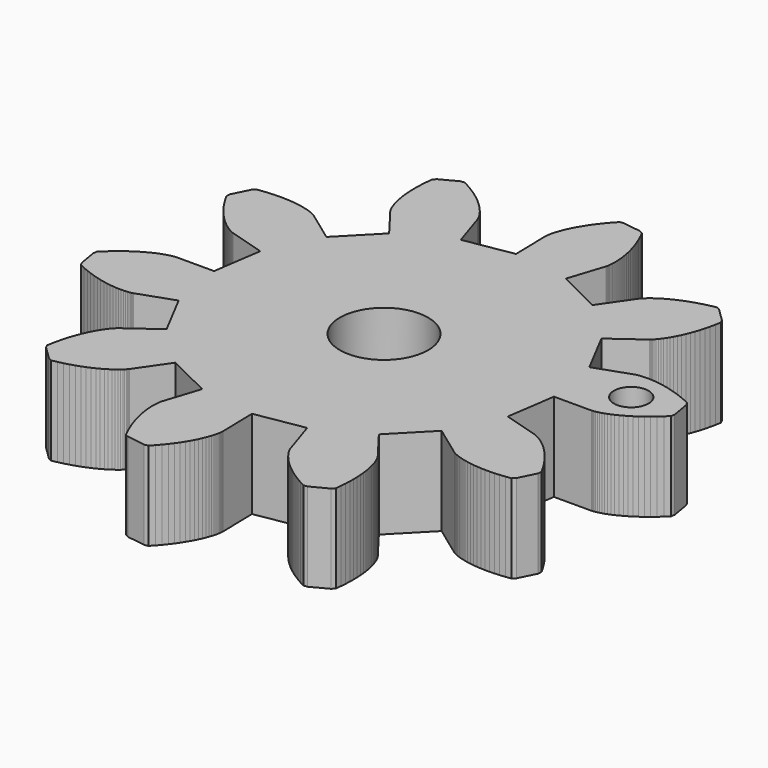
from build123d import *

# Parameters (mm, degrees)
F0_R     = 2.5
F1_DEPTH = 5


# Not quite as in the source:
# - the dataset's text gives a spline's control points without its knots; the knots are read off the source's solid


with BuildPart() as f1:
    # F0 (on Top) → F1 (new body)
    with BuildSketch(Plane.XY):
        Polygon((13.6310377596, 0.7067476629), (14.0365257596, 3.4714366629), (16.1597377596, 3.4714366629), (16.1738627596, 3.4719536629), (16.2024577596, 3.4740206629), (16.2451767596, 3.4784996629), (16.3016757596, 3.4865956629), (16.3723007596, 3.4989976629), (16.4563607596, 3.5169126629), (16.5535127596, 3.5412006629), (16.6634107596, 3.5727226629), (16.7860567596, 3.6126856629), (16.9204147596, 3.6616066629), (17.0664877596, 3.7206896629), (17.2232387596, 3.7906246629), (17.3903257596, 3.8721016629), (17.5674037596, 3.9661526629), (17.7530947596, 4.0736396629), (17.9473977596, 4.1949066629), (18.1492807596, 4.3309886629), (18.3573647596, 4.4825726629), (18.5716497596, 4.6500046629), (18.7911017596, 4.8339726629), (19.0143447596, 5.0351656629), (19.2406867596, 5.2539296629), (19.2785827596, 5.4651136629), (19.1015047596, 6.5055326629), (18.9960847596, 6.6924286629), (18.7101427596, 6.8238596629), (18.4328117596, 6.9399586629), (18.1651277596, 7.0410726629), (17.9074347596, 7.1282336629), (17.6607657596, 7.2023036629), (17.4254657596, 7.2641426629), (17.2018797596, 7.3144406629), (16.9910397596, 7.3542316629), (16.7929467596, 7.3845486629), (16.6082897596, 7.4064246629), (16.4370687596, 7.4203776629), (16.2799717596, 7.4277846629), (16.1366557596, 7.4296796629), (16.0078097596, 7.4267506629), (15.8937767596, 7.4202056629), (15.7938687596, 7.4109036629), (15.7087747596, 7.4000516629), (15.6381507596, 7.3885106629), (15.5819957596, 7.3773136629), (15.5399657596, 7.3674956629), (15.5124047596, 7.3599166629), (15.4989687596, 7.3557826629), (13.4953017596, 6.6538436629), (12.1985677596, 9.1289726629), (13.9159477596, 10.3767866629), (13.9273167596, 10.3855716629), (13.9490207596, 10.4040026629), (13.9810597596, 10.4327696629), (14.0220567596, 10.4725596629), (14.0716657596, 10.5240646629), (14.1291987596, 10.5879706629), (14.1936217596, 10.6646236629), (14.2639017596, 10.7548856629), (14.3396937596, 10.8590996629), (14.4196207596, 10.9777836629), (14.5029917596, 11.1112806629), (14.5887747596, 11.2601086629), (14.6762797596, 11.4244396629), (14.7641297596, 11.6044466629), (14.8512907596, 11.8006446629), (14.9370737596, 12.0130346629), (15.0201007596, 12.2416166629), (15.0996827596, 12.4865626629), (15.1747857596, 12.7480456629), (15.2436867596, 13.0257206629), (15.3063877596, 13.3197596629), (15.3608207596, 13.6298176629), (15.2674587596, 13.8229156629), (14.5126377596, 14.5606826629), (14.3176457596, 14.6497386629), (14.0086207596, 14.5880706629), (13.7161317596, 14.5189966629), (13.4401797596, 14.4433766629), (13.1804197596, 14.3625896629), (12.9375407596, 14.2773236629), (12.7108527596, 14.1891286629), (12.5003577596, 14.0985226629), (12.3063987596, 14.0067116629), (12.1282877596, 13.9148996629), (11.9660237596, 13.8237766629), (11.8192627596, 13.7345486629), (11.6876597596, 13.6482486629), (11.5708707596, 13.5655666629), (11.4682067596, 13.4875356629), (11.3796677596, 13.4150156629), (11.3045647596, 13.3488706629), (11.2418647596, 13.2899586629), (11.1915657596, 13.2391436629), (11.1526367596, 13.1971136629), (11.1247307596, 13.1645576629), (11.1068167596, 13.1423366629), (11.0982037596, 13.1307956629), (9.8900087596, 11.3853376629), (7.3857687596, 12.6254006629), (8.0420597596, 14.6443986629), (8.0458487596, 14.6581786629), (8.0527397596, 14.6859116629), (8.0616967596, 14.7279416629), (8.0716877596, 14.7844416629), (8.0813337596, 14.8552386629), (8.0902907596, 14.9406766629), (8.0971807596, 15.0405846629), (8.1013157596, 15.1549616629), (8.1013157596, 15.2838086629), (8.0961477596, 15.4267796629), (8.0851237596, 15.5838756629), (8.0672087596, 15.7545806629), (8.0413707596, 15.9388926629), (8.0062307596, 16.1362966629), (7.9617887596, 16.3461036629), (7.9063227596, 16.5683116629), (7.8391437596, 16.8022336629), (7.7595617596, 17.0471806629), (7.6665437596, 17.3028066629), (7.5590577596, 17.5680786629), (7.4371007596, 17.8426526629), (7.2989527596, 18.1254956629), (7.1098167596, 18.2267806629), (6.0656087596, 18.3800876629), (5.8551127596, 18.3373686629), (5.6415167596, 18.1060306629), (5.4458357596, 17.8781376629), (5.2666907596, 17.6547226629), (5.1040817596, 17.4368206629), (4.9576657596, 17.2249476629), (4.8260627596, 17.0203086629), (4.7092747596, 16.8232486629), (4.6059217596, 16.6351466629), (4.5160047596, 16.4560016629), (4.4381457596, 16.2870196629), (4.3719997596, 16.1285456629), (4.3161887596, 15.9814396629), (4.2703687596, 15.8458756629), (4.2333347596, 15.7223686629), (4.2042237596, 15.6117816629), (4.1821747596, 15.5139406629), (4.1663267596, 15.4295356629), (4.1553027596, 15.3589116629), (4.1487567596, 15.3020676629), (4.1451397596, 15.2591756629), (4.1437617596, 15.2305816629), (4.1435897596, 15.2162846629), (4.1919927596, 13.0939336629), (1.4372947596, 12.6254006629), (0.7813487596, 14.6443986629), (0.7763537596, 14.6578346629), (0.7656737596, 14.6843616629), (0.7481037596, 14.7234636629), (0.7229547596, 14.7749676629), (0.6893647596, 14.8381846629), (0.6463007596, 14.9125986629), (0.5932467596, 14.9973486629), (0.5291677596, 15.0922606629), (0.4533757596, 15.1964746629), (0.3653537596, 15.3093016629), (0.2640677596, 15.4298806629), (0.1491737596, 15.5575206629), (0.0198107596, 15.6911906629), (-0.1243672404, 15.8303726629), (-0.2838752404, 15.9740326629), (-0.4594022404, 16.1211386629), (-0.6511222404, 16.2710006629), (-0.8595502404, 16.4222396629), (-1.0850322404, 16.5743406629), (-1.3277392404, 16.7259246629), (-1.5880162404, 16.8763036629), (-1.8660352404, 17.0239256629), (-2.0785972404, 16.9946426629), (-3.0134242404, 16.5049226629), (-3.1584622404, 16.3467926629), (-3.1953252404, 16.0339776629), (-3.2199572404, 15.7345986629), (-3.2333932404, 15.4486556629), (-3.2366662404, 15.1766656629), (-3.2308092404, 14.9191446629), (-3.2168572404, 14.6762656629), (-3.1956692404, 14.4482006629), (-3.1684532404, 14.2352936629), (-3.1360692404, 14.0375446629), (-3.0997232404, 13.8551266629), (-3.0601052404, 13.6880396629), (-3.0185912404, 13.5361116629), (-2.9760442404, 13.3995136629), (-2.9334982404, 13.2779016629), (-2.8919842404, 13.1712756629), (-2.8523662404, 13.0792916629), (-2.8156752404, 13.0016046629), (-2.7829472404, 12.9380426629), (-2.7548692404, 12.8880886629), (-2.7326482404, 12.8513986629), (-2.7169732404, 12.8272826629), (-2.7087052404, 12.8157416629), (-1.4221342404, 11.1271286629), (-3.3751592404, 9.1289726629), (-5.0927112404, 10.3767866629), (-5.1045972404, 10.3847096629), (-5.1288852404, 10.3998686629), (-5.1660922404, 10.4212276629), (-5.2167352404, 10.4480996629), (-5.2809862404, 10.4794506629), (-5.3595342404, 10.5142456629), (-5.4523792404, 10.5517976629), (-5.5598662404, 10.5908986629), (-5.6825122404, 10.6306896629), (-5.8199712404, 10.6701366629), (-5.9727612404, 10.7082046629), (-6.1408812404, 10.7436886629), (-6.3239882404, 10.7760726629), (-6.5224262404, 10.8039786629), (-6.7360222404, 10.8263716629), (-6.9644322404, 10.8422186629), (-7.2074832404, 10.8506596629), (-7.4651762404, 10.8506596629), (-7.7369942404, 10.8411856629), (-8.0224202404, 10.8212036629), (-8.3212822404, 10.7896806629), (-8.6330642404, 10.7457556629), (-8.7879212404, 10.5971006629), (-9.2562812404, 9.6514216629), (-9.2807412404, 9.4381696629), (-9.1265732404, 9.1635956629), (-8.9705112404, 8.9067646629), (-8.8134142404, 8.6675026629), (-8.6561462404, 8.4456376629), (-8.5000832404, 8.2406546629), (-8.3459152404, 8.0523806629), (-8.1948472404, 7.8804706629), (-8.0475702404, 7.7240626629), (-7.9052872404, 7.5831586629), (-7.7685172404, 7.4570676629), (-7.6382922404, 7.3451026629), (-7.5154752404, 7.2465726629), (-7.4007532404, 7.1609616629), (-7.2948162404, 7.0877536629), (-7.1985262404, 7.0257416629), (-7.1123982404, 6.9745826629), (-7.0371232404, 6.9334136629), (-6.9732172404, 6.9012016629), (-6.9211962404, 6.8772586629), (-6.8815772404, 6.8607216629), (-6.8548772404, 6.8505586629), (-6.8412692404, 6.8459076629), (-4.8078022404, 6.2361256629), (-5.2134622404, 3.4714366629), (-7.3363302404, 3.4714366629), (-7.3506272404, 3.4709206629), (-7.3792212404, 3.4688536629), (-7.4219402404, 3.4642026629), (-7.4786122404, 3.4562786629), (-7.5490642404, 3.4438766629), (-7.6329522404, 3.4259616629), (-7.7302762404, 3.4016736629), (-7.8403472404, 3.3699786629), (-7.9628202404, 3.3301876629), (-8.0971792404, 3.2812676629), (-8.2432512404, 3.2223566629), (-8.4000032404, 3.1524216629), (-8.5672622404, 3.0707726629), (-8.7441682404, 2.9767216629), (-8.9300312404, 2.8692346629), (-9.1241622404, 2.7479666629), (-9.3258722404, 2.6118856629), (-9.5343012404, 2.4603016629), (-9.7484132404, 2.2928696629), (-9.9676942404, 2.1089016629), (-10.1911082404, 1.9077086629), (-10.4174512404, 1.6889446629), (-10.4553472404, 1.4777606629), (-10.2782692404, 0.4373416629), (-10.1728492404, 0.2506176629), (-9.8867342404, 0.1190146629), (-9.6095762404, 0.0029146629), (-9.3417202404, -0.0983713371), (-9.0841992404, -0.1855323371), (-8.8375302404, -0.2596013371), (-8.6022302404, -0.3212683371), (-8.3788152404, -0.3715673371), (-8.1678032404, -0.4115303371), (-7.9697102404, -0.4418473371), (-7.7850532404, -0.4635513371), (-7.6138322404, -0.4776763371), (-7.4565632404, -0.4849103371), (-7.3134202404, -0.4866333371), (-7.1847452404, -0.4838773371), (-7.0703682404, -0.4773313371), (-6.9706332404, -0.4680293371), (-6.8855392404, -0.4573503371), (-6.8149142404, -0.4456363371), (-6.7587592404, -0.4346123371), (-6.7169012404, -0.4246213371), (-6.6893412404, -0.4170423371), (-6.6755602404, -0.4129083371), (-4.6720652404, 0.2888576629), (-3.3751592404, -2.1860983371), (-5.0927112404, -3.4339123371), (-5.1039082404, -3.4428693371), (-5.1257842404, -3.4611283371), (-5.1576512404, -3.4897233371), (-5.1988202404, -3.5296863371), (-5.2486022404, -3.5813623371), (-5.3059632404, -3.6450963371), (-5.3703862404, -3.7219223371), (-5.4408382404, -3.8121843371), (-5.5164582404, -3.9162253371), (-5.5963842404, -4.0350813371), (-5.6797552404, -4.1684063371), (-5.7657112404, -4.3172353371), (-5.8530442404, -4.4815663371), (-5.9407212404, -4.6617443371), (-6.0280552404, -4.8577703371), (-6.1138372404, -5.0699883371), (-6.1970372404, -5.2987423371), (-6.2766182404, -5.5436893371), (-6.3515492404, -5.8051713371), (-6.4206232404, -6.0828463371), (-6.4831522404, -6.3767133371), (-6.5377562404, -6.6867713371), (-6.4442222404, -6.8800413371), (-5.6894022404, -7.6176363371), (-5.4942372404, -7.7068643371), (-5.1855562404, -7.6451973371), (-4.8930682404, -7.5759503371), (-4.6169432404, -7.5005033371), (-4.3573562404, -7.4195433371), (-4.1141322404, -7.3344493371), (-3.8874442404, -7.2462553371), (-3.6771212404, -7.1556493371), (-3.4831632404, -7.0640093371), (-3.3050512404, -6.9720253371), (-3.1427872404, -6.8810753371), (-2.9960262404, -6.7918473371), (-2.8644232404, -6.7053753371), (-2.7476352404, -6.6226923371), (-2.6451432404, -6.5444893371), (-2.5566042404, -6.4721423371), (-2.4813292404, -6.4059963371), (-2.4186282404, -6.3470853371), (-2.3683302404, -6.2964423371), (-2.3295722404, -6.2544123371), (-2.3014952404, -6.2216833371), (-2.2835802404, -6.1992903371), (-2.2749682404, -6.1879213371), (-1.0666002404, -4.4422913371), (1.4372947596, -5.6825263371), (0.7813487596, -7.7016963371), (0.7773867596, -7.7154773371), (0.7704967596, -7.7430373371), (0.7615397596, -7.7850683371), (0.7517207596, -7.8415673371), (0.7419027596, -7.9125363371), (0.7329447596, -7.9976303371), (0.7258827596, -8.0975383371), (0.7219207596, -8.2122593371), (0.7220927596, -8.3411063371), (0.7270887596, -8.4840783371), (0.7381127596, -8.6408293371), (0.7560267596, -8.8117063371), (0.7820377596, -8.9960193371), (0.8168327596, -9.1934233371), (0.8614467596, -9.4032293371), (0.9169127596, -9.6254383371), (0.9840927596, -9.8593603371), (1.0636737596, -10.1043063371), (1.1566917596, -10.3599323371), (1.2640067596, -10.6252043371), (1.3863077596, -10.8997783371), (1.5242837596, -11.1826213371), (1.7135917596, -11.2839073371), (2.7577997596, -11.4372133371), (2.9681227596, -11.3944943371), (3.1815467596, -11.1633283371), (3.3775727596, -10.9352633371), (3.5565457596, -10.7120213371), (3.7189817596, -10.4939463371), (3.8657427596, -10.2820733371), (3.9971727596, -10.0774343371), (4.1141337596, -9.8803753371), (4.2171427596, -9.6922723371), (4.3072317596, -9.5131283371), (4.3850907596, -9.3443183371), (4.4512367596, -9.1858433371), (4.5070467596, -9.0383933371), (4.5528667596, -8.9030013371), (4.5897297596, -8.7796673371), (4.6190127596, -8.6687353371), (4.6410617596, -8.5712383371), (4.6569087596, -8.4868343371), (4.6679327596, -8.4158653371), (4.6744787596, -8.3590213371), (4.6782687596, -8.3163013371), (4.6793017596, -8.2877073371), (4.6796467596, -8.2735823371), (4.6314147596, -6.1510593371), (7.3857687596, -5.6825263371), (8.0420597596, -7.7016963371), (8.0468827596, -7.7151323371), (8.0575627596, -7.7416593371), (8.0751327596, -7.7805893371), (8.1002817596, -7.8322653371), (8.1340437596, -7.8953113371), (8.1767627596, -7.9697253371), (8.2301617596, -8.0544743371), (8.2938957596, -8.1495593371), (8.3696877596, -8.2536013371), (8.4578827596, -8.3662553371), (8.5591687596, -8.4868343371), (8.6742347596, -8.6146473371), (8.8034257596, -8.7483163371), (8.9474307596, -8.8874983371), (9.1072827596, -9.0311593371), (9.2826387596, -9.1782643371), (9.4741857596, -9.3281263371), (9.6826137596, -9.4793663371), (9.9082677596, -9.6316393371), (10.1508027596, -9.7832233371), (10.4112517596, -9.9334293371), (10.6892707596, -10.0812243371), (10.9018337596, -10.0519403371), (11.8364877596, -9.5620483371), (11.9818707596, -9.4039183371), (12.0183887596, -9.0911033371), (12.0431937596, -8.7917253371), (12.0566297596, -8.5057823371), (12.0597297596, -8.2339643371), (12.0542177596, -7.9762703371), (12.0400927596, -7.7333913371), (12.0190777596, -7.5053263371), (11.9915167596, -7.2924193371), (11.9594777596, -7.0946703371), (11.9229597596, -6.9124253371), (11.8833407596, -6.7449933371), (11.8419997596, -6.5934093371), (11.7992807596, -6.4566393371), (11.7569057596, -6.3350273371), (11.7152207596, -6.2282293371), (11.6756017596, -6.1362453371), (11.6390837596, -6.0587303371), (11.6060107596, -5.9949963371), (11.5781057596, -5.9450423371), (11.5560567596, -5.9085243371), (11.5402097596, -5.8844083371), (11.5319417596, -5.8726953371), (10.2451977596, -4.1842543371), (12.1985677596, -2.1860983371), (13.9159477596, -3.4339123371), (13.9276607596, -3.4418363371), (13.9521207596, -3.4569943371), (13.9893277596, -3.4783543371), (14.0399707596, -3.5052263371), (14.1040497596, -3.5365763371), (14.1825977596, -3.5713713371), (14.2756157596, -3.6089233371), (14.3831027596, -3.6481973371), (14.5057477596, -3.6878163371), (14.6432067596, -3.7270903371), (14.7961697596, -3.7653303371), (14.9639457596, -3.8008153371), (15.1472247596, -3.8331993371), (15.3456617596, -3.8611043371), (15.5592577596, -3.8834973371), (15.7876677596, -3.8993443371), (16.0308917596, -3.9079573371), (16.2882397596, -3.9076133371), (16.5600577596, -3.8983113371), (16.8456567596, -3.8783293371), (17.1446907596, -3.8466343371), (17.4564717596, -3.8028823371), (17.6111567596, -3.6543983371), (18.0793457596, -2.7083753371), (18.1038057596, -2.4954683371), (17.9498097596, -2.2208943371), (17.7937467596, -1.9638903371), (17.6366507596, -1.7248003371), (17.4795537596, -1.5025923371), (17.3231467596, -1.2979533371), (17.1691507596, -1.1095063371), (17.0182557596, -0.9375963371), (16.8708057596, -0.7811893371), (16.7285237596, -0.6402843371), (16.5917527596, -0.5141943371), (16.4615287596, -0.4022283371), (16.3385387596, -0.3036983371), (16.2238167596, -0.2182603371), (16.1180527596, -0.1448793371), (16.0215897596, -0.0828683371), (15.9354627596, -0.0318803371), (15.8603597596, 0.0094606629), (15.7962807596, 0.0414996629), (15.7442597596, 0.0656156629), (15.7049857596, 0.0821516629), (15.6781137596, 0.0924876629), (15.6646777596, 0.0969656629), align=None)
        with Locations((4.4117037596, 3.4714366629)):
            Circle(F0_R, mode=Mode.SUBTRACT)
        with BuildLine():
            add(Edge.make_bspline(
                [(17.7158877596, 5.5676056629), (17.7158877596, 6.1095186629), (17.2766377596, 6.5489406629), (16.7347247596, 6.5489406629), (16.1928107596, 6.5489406629), (15.7532167596, 6.1095186629), (15.7532167596, 5.5676056629), (15.7532167596, 5.0256916629), (16.1928107596, 4.5862696629), (16.7347247596, 4.5862696629), (17.2766377596, 4.5862696629), (17.7158877596, 5.0256916629), (17.7158877596, 5.5676056629)],
                knots=[0, 0, 0, 0, 1, 1, 1, 2, 2, 2, 3, 3, 3, 4, 4, 4, 4], degree=3))
        make_face(mode=Mode.SUBTRACT)
    extrude(amount=F1_DEPTH)


solid = f1.part
